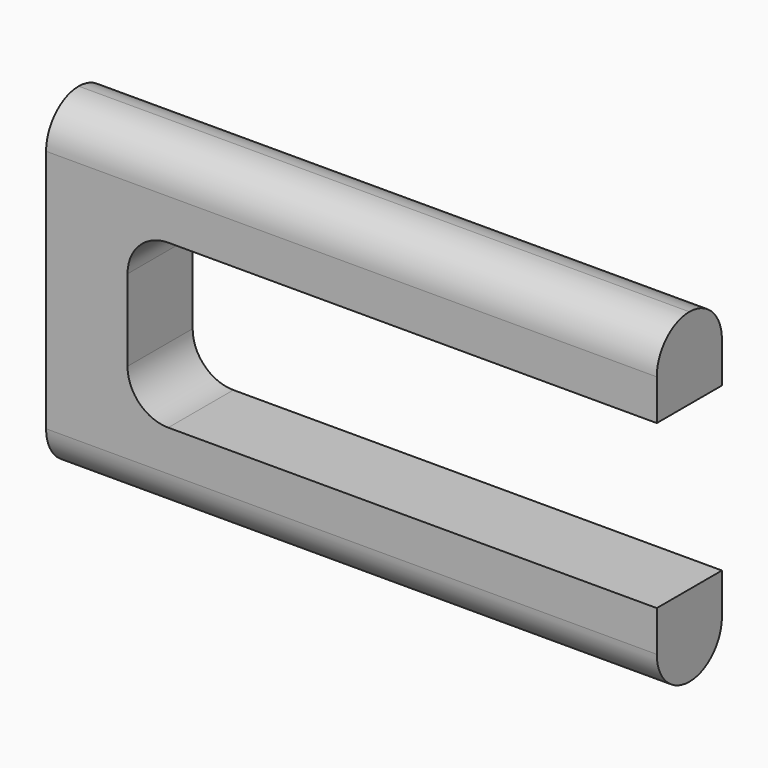
from build123d import *

# Parameters (mm, degrees)
F1_DEPTH = 2
F2_R     = 1.99999


# Not quite as in the source:
# - a fillet or chamfer is up to 0.001 mm smaller than in the source, because OpenCascade refuses the exact size


with BuildPart() as f1:
    # F0 (on Front) → F1 (new body, symmetric)
    with BuildSketch(Plane.XZ):
        Polygon((0, 12), (0, 16), (-30, 16), (-30, 0), (0, 0), (0, 4), (-26, 4), (-26, 12), align=None)
    extrude(amount=F1_DEPTH, both=True)

    # F2 (radius 2 in the source; OpenCascade refuses exactly that, so slightly less here)
    f2_edges = [f1.edges().sort_by_distance(p)[0] for p in [
        (-15, -2, 16),
        (-15, 2, 16),
        (-15, -2, 0),
        (-15, 2, 0),
        (-26, 0, 4),
        (-26, 0, 12),
    ]]
    fillet(f2_edges, radius=F2_R)


solid = f1.part
